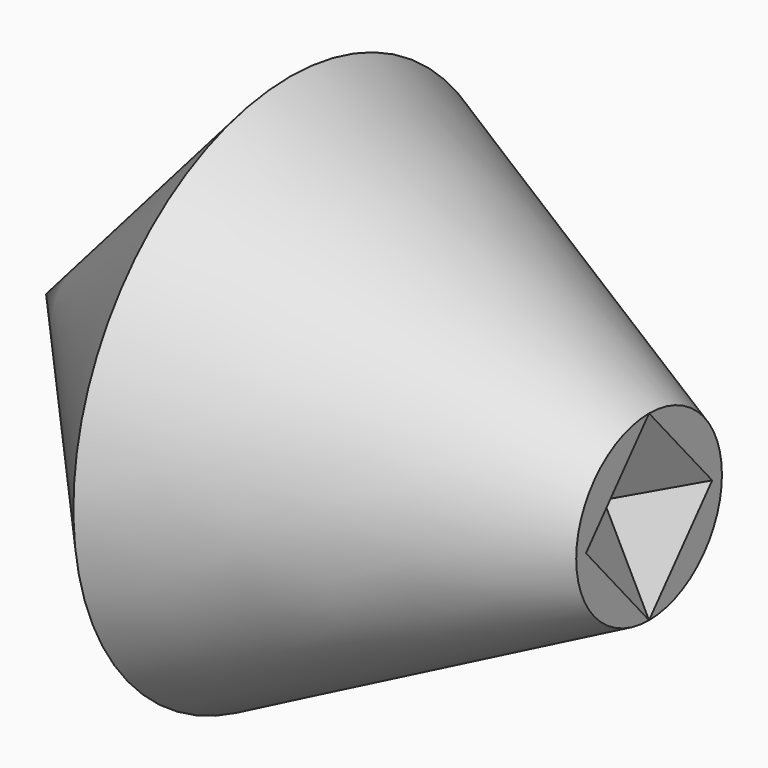
from build123d import *


with BuildPart() as f1:
    # F0 (on Front) → F1 (revolve)
    with BuildSketch(Plane.XZ):
        Polygon((-6.35, 0), (-6.35, 12.7), (-12.7, 0), align=None)
        Polygon((-12.7, 0), (-6.35, 12.7), (-56.4411745648, 37.7455872824), (-90.4398604321, 0), align=None)
    revolve(axis=Axis((-6.35, 0, 0), (1, 0, 0)))

    # F2 (on Top) → F7 section 0
    with BuildSketch(Plane.XY, mode=Mode.PRIVATE) as f7_s0:
        Polygon((-6.35, -10.9985226281), (6.35, -10.9985226281), (12.7, 0), (6.35, 10.9985226281), (-6.35, 10.9985226281), (-12.7, 0), align=None)
    loft([Vertex(0, 0, -25.4), f7_s0.sketch], mode=Mode.SUBTRACT)

    # F2 (on Top) → F8 section 0
    with BuildSketch(Plane.XY, mode=Mode.PRIVATE) as f8_s0:
        Polygon((-6.35, -10.9985226281), (6.35, -10.9985226281), (12.7, 0), (6.35, 10.9985226281), (-6.35, 10.9985226281), (-12.7, 0), align=None)
    loft([Vertex(0, 0, 25.4), f8_s0.sketch], mode=Mode.SUBTRACT)


solid = f1.part
